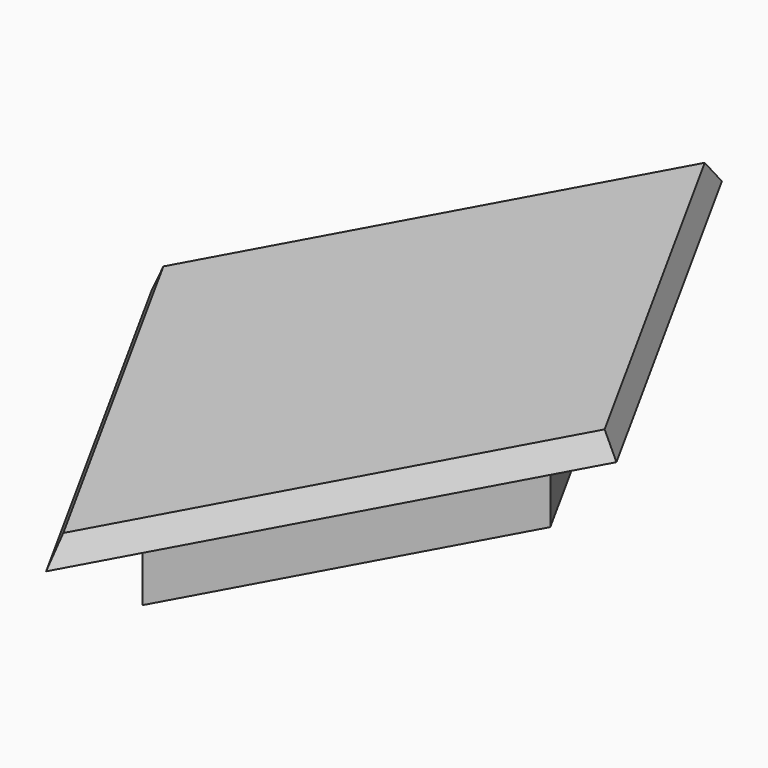
from build123d import *

# Parameters (mm, degrees)
F1_DEPTH = 34.925
F2_DEPTH = 11.1125
F3_SIZE2 = 11.11249
F3_SIZE  = 4.602938


# Not quite as in the source:
# - a fillet or chamfer is up to 0.001 mm smaller than in the source, because OpenCascade refuses the exact size


with BuildPart() as f1:
    # F0 (on Top) → F1 (new body)
    with BuildSketch(Plane.XY):
        Polygon((0, -134.14375), (0, 134.14375), (-73.81875, 0), align=None)
        Polygon((73.81875, 0), (0, 134.14375), (0, -134.14375), align=None)
    extrude(amount=-F1_DEPTH)

    # F0 (on Top) + F1_face (on face) → F2 (join)
    with BuildSketch(Plane.XY):
        Polygon((-103.1875, 0), (0, -187.5127688172), (103.1875, 0), (0, 187.5127688172), align=None)
        Polygon((-73.81875, 0), (0, 134.14375), (73.81875, 0), (0, -134.14375), align=None, mode=Mode.SUBTRACT)
    with BuildSketch(Plane.XY):
        Polygon((0, 134.14375), (-73.81875, 0), (0, -134.14375), (73.81875, 0), align=None)
    extrude(amount=F2_DEPTH)

    # F3 (size 4.6029482119 and 11.1125 in the source; OpenCascade refuses exactly that, so slightly less here)
    f3_edges = [f1.edges().sort_by_distance(p)[0] for p in [
        (-51.59375, -93.756384, 11.1125),
        (-51.59375, 93.756384, 11.1125),
        (51.59375, 93.756384, 11.1125),
        (51.59375, -93.756384, 11.1125),
    ]]
    f3_side = f1.faces().sort_by_distance((0, 0, 11.1125))[0]
    chamfer(f3_edges, length=F3_SIZE, length2=F3_SIZE2, reference=f3_side)


solid = f1.part
